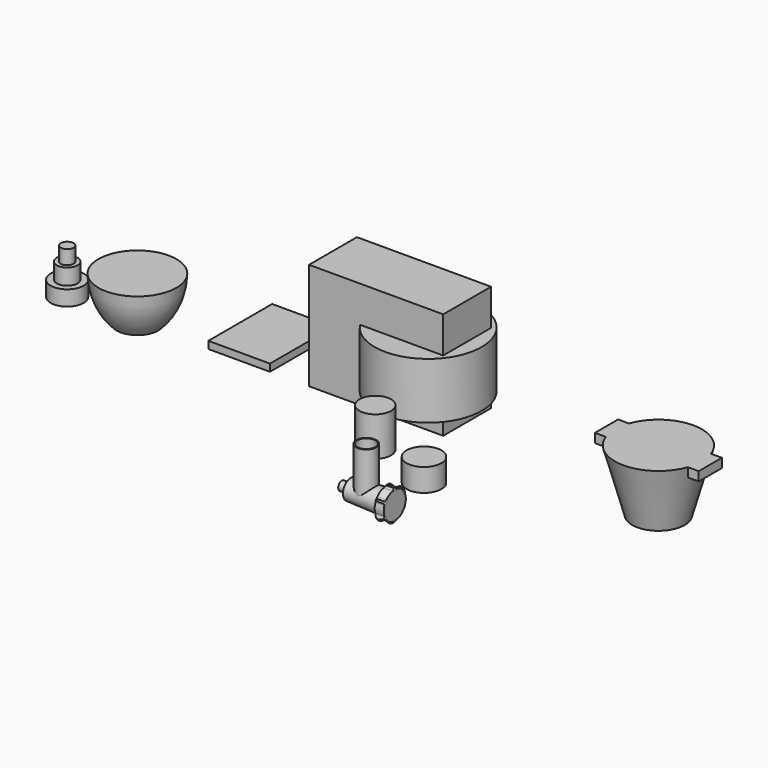
from build123d import *

# Parameters (mm, degrees)
F0_W          = 170
F0_H          = 220
F1_DEPTH      = 20
F2_W          = 370
F2_H          = 165
F3_DEPTH      = 40
F5_DEPTH      = 155
F6_W          = 370
F6_H          = 165
F7_DEPTH      = 100
F10_W         = 30
F10_H         = 80
F11_DEPTH     = 25
F12_R         = 43.5
F13_DEPTH     = 108
F14_R         = 48
F15_DEPTH     = 63
F16_R         = 27.5
F19_R         = 31
F22_DEPTH     = 25
F23_R         = 12.49999
F24_T4_DEPTH  = 46.1160280669
F24_S5_R      = 12.49999
F24_T6_DEPTH  = 25
F24_T10_DEPTH = 46.1160280669
F24_S11_R     = 12.49999
F24_T12_DEPTH = 25
F24_T16_DEPTH = 46.1160280669
F24_S17_R     = 12.49999
F24_T18_DEPTH = 25
F24_T22_DEPTH = 46.1160280669
F24_S23_R     = 12.49999
F24_T24_DEPTH = 25
F24_T28_DEPTH = 46.1160280669
F24_S29_R     = 12.49999
F24_T30_DEPTH = 25
F24_T34_DEPTH = 46.1160280669
F24_S35_R     = 12.49999
F24_T36_DEPTH = 25
F24_T40_DEPTH = 46.1160280669
F24_S41_R     = 12.49999
F24_T42_DEPTH = 25
F24_T46_DEPTH = 46.1160280669
F24_S47_R     = 12.49999
F24_T48_DEPTH = 25
F24_T52_DEPTH = 46.1160280669
F24_S53_R     = 12.49999
F24_T54_DEPTH = 25
F24_T58_DEPTH = 46.1160280669
F24_S59_R     = 12.49999
F24_T60_DEPTH = 25
F24_T64_DEPTH = 46.1160280669
F24_S65_R     = 12.49999
F24_T66_DEPTH = 25
F24_T70_DEPTH = 46.1160280669
F24_S71_R     = 12.49999
F24_T72_DEPTH = 25
F25_R         = 12.5
F26_DEPTH     = 25
F27_R         = 27.5
F27_R_2       = 25
F28_DEPTH     = 124


# Not quite as in the source:
# - a fillet or chamfer that OpenCascade refuses, or shapes differently, is made with other operations: its cross-section is extruded or revolved along the edge and cut away or added
# - a fillet or chamfer is up to 0.001 mm smaller than in the source, because OpenCascade refuses the exact size


with BuildPart() as f1:
    # F0 (on Top) → F1 (new body)
    with BuildSketch(Plane.XY):
        with Locations((-562.7675076718, 110)):
            Rectangle(F0_W, F0_H)
    extrude(amount=F1_DEPTH)


with BuildPart() as f3:
    # F2 (on Top) → F3 (new body)
    with BuildSketch(Plane.XY):
        with Locations((-185, 82.5)):
            Rectangle(F2_W, F2_H)
    extrude(amount=F3_DEPTH)

    # F4 (on face) → F5 (join)
    with BuildSketch(Plane.XY.offset(40)):
        with BuildLine():
            Line((-370, 0), (-229.7701926064, 0))
            ThreePointArc((-229.7701926064, 0), (40, 82.5), (-229.7701926064, 165))
            Line((-229.7701926064, 165), (-370, 165))
            Line((-370, 165), (-370, 0))
        make_face()
    extrude(amount=F5_DEPTH)

    # F6 (on face) → F7 (join)
    with BuildSketch(Plane.XY.offset(195)):
        with Locations((-185, 82.5)):
            Rectangle(F6_W, F6_H)
    extrude(amount=F7_DEPTH)


with BuildPart() as f9:
    # F8 (on Front) → F9 (revolve)
    with BuildSketch(Plane.XZ):
        Polygon((593.6409032087, 170), (593.6409032087, 0), (666.1409032087, 0), (713.6409032087, 170), align=None)
    revolve(axis=Axis((593.6409032087, 0, 85), (0, 0, 1)))

    # F10 (on face) → F11 (join)
    with BuildSketch(Plane.XY.offset(170)):
        with Locations((465.5038182188, 0)):
            Rectangle(F10_W, F10_H)
        with Locations((721.7779881985, 0)):
            Rectangle(F10_W, F10_H)
    extrude(amount=-F11_DEPTH)


with BuildPart() as f13:
    # F12 (on Top) → F13 (new body)
    with BuildSketch(Plane.XY):
        with Locations((-74.1944685578, -141.4187550545)):
            Circle(F12_R)
    extrude(amount=F13_DEPTH)


with BuildPart() as f15:
    # F14 (on Top) → F15 (new body)
    with BuildSketch(Plane.XY):
        with Locations((104.2551547289, -196.5236961842)):
            Circle(F14_R)
    extrude(amount=F15_DEPTH)


with BuildPart() as f20:
    # F16 (on Right) → F20 section 0
    with BuildSketch(Plane.YZ):
        with Locations((-318.2184583697, 0)):
            Circle(F16_R)
    # F19 (on offset) → F20 section 1
    with BuildSketch(Plane.YZ.offset(96)):
        with Locations((-318.2184583697, 0)):
            Circle(F19_R)
    loft()

    # F21 (on face) → F22 (join)
    with BuildSketch(Plane.YZ.offset(96)):
        with BuildLine():
            Line((-320.7184583697, 46.9176739793), (-320.7184583697, 37.9176739793))
            ThreePointArc((-320.7184583697, 37.9176739793), (-337.2184583697, 32.9089653438), (-349.8061272882, 21.1239004991))
            Line((-349.8061272882, 21.1239004991), (-357.6003559222, 25.6239004991))
            Line((-357.6003559222, 25.6239004991), (-360.1003559222, 21.2937734802))
            Line((-360.1003559222, 21.2937734802), (-352.3061272882, 16.7937734802))
            ThreePointArc((-352.3061272882, 16.7937734802), (-356.2184583697, 0), (-352.3061272882, -16.7937734802))
            Line((-352.3061272882, -16.7937734802), (-360.1003559222, -21.2937734802))
            Line((-360.1003559222, -21.2937734802), (-357.6003559222, -25.6239004991))
            Line((-357.6003559222, -25.6239004991), (-349.8061272882, -21.1239004991))
            ThreePointArc((-349.8061272882, -21.1239004991), (-337.2184583697, -32.9089653438), (-320.7184583697, -37.9176739793))
            Line((-320.7184583697, -37.9176739793), (-320.7184583697, -46.9176739793))
            Line((-320.7184583697, -46.9176739793), (-315.7184583697, -46.9176739793))
            Line((-315.7184583697, -46.9176739793), (-315.7184583697, -37.9176739793))
            ThreePointArc((-315.7184583697, -37.9176739793), (-299.2184583697, -32.9089653438), (-286.6307894512, -21.1239004991))
            Line((-286.6307894512, -21.1239004991), (-278.8365608172, -25.6239004991))
            Line((-278.8365608172, -25.6239004991), (-276.3365608172, -21.2937734802))
            Line((-276.3365608172, -21.2937734802), (-284.1307894512, -16.7937734802))
            ThreePointArc((-284.1307894512, -16.7937734802), (-280.2184583697, 0), (-284.1307894512, 16.7937734802))
            Line((-284.1307894512, 16.7937734802), (-276.3365608172, 21.2937734802))
            Line((-276.3365608172, 21.2937734802), (-278.8365608172, 25.6239004991))
            Line((-278.8365608172, 25.6239004991), (-286.6307894512, 21.1239004991))
            ThreePointArc((-286.6307894512, 21.1239004991), (-299.2184583697, 32.9089653438), (-315.7184583697, 37.9176739793))
            Line((-315.7184583697, 37.9176739793), (-315.7184583697, 46.9176739793))
            Line((-315.7184583697, 46.9176739793), (-320.7184583697, 46.9176739793))
        make_face()
    extrude(amount=F22_DEPTH)

    # F23 (radius 12.5 in the source; OpenCascade refuses exactly that, so slightly less here)
    f23_edges = [f20.edges().sort_by_distance(p)[0] for p in [
        (96, -358.850356, 23.458837),
        (121, -358.850356, 23.458837),
        (96, -358.850356, -23.458837),
        (121, -358.850356, -23.458837),
        (121, -318.218458, -46.917674),
        (96, -318.218458, -46.917674),
        (96, -277.586561, -23.458837),
        (121, -277.586561, -23.458837),
        (96, -277.586561, 23.458837),
        (121, -277.586561, 23.458837),
        (96, -318.218458, 46.917674),
        (121, -318.218458, 46.917674),
    ]]
    fillet(f23_edges, radius=F23_R)

    # F24: fillet of radius 5 on 12 edges, made by hand


with BuildPart() as f24_tool2:
    # F24_s3 → F24_t4 (new body)
    with BuildSketch(Plane.YZ.offset(85.4419859665)):
        with BuildLine():
            ThreePointArc((-353.9369352588, -12.9688244926), (-353.9389410675, -16.3871873128), (-356.1367348495, -19.0053757869))
            Line((-356.1367348495, -19.0053757869), (-352.3061272882, -16.7937734802))
            ThreePointArc((-352.3061272882, -16.7937734802), (-353.1738879454, -14.9036218142), (-353.9369352588, -12.9688244926))
        make_face()
    extrude(amount=F24_T4_DEPTH)

    # F24_s5 → F24_t6 (intersect, symmetric)
    with BuildSketch(Plane(origin=(0, -81.65, 141.421948438), x_dir=(1, 0, 0), z_dir=(0, 0.5, -0.8660254038))):
        with Locations((108.50001, 310.0029528806)):
            Circle(F24_S5_R)
    extrude(amount=F24_T6_DEPTH, both=True, mode=Mode.INTERSECT)


with BuildPart() as f20_1:
    add(f20.part)

    # F24_t1: union F24_tool2
    add(f24_tool2.part)


with BuildPart() as f24_tool8:
    # F24_s9 → F24_t10 (new body)
    with BuildSketch(Plane.YZ.offset(85.4419859665)):
        with BuildLine():
            ThreePointArc((-353.9369352588, 12.9688244926), (-353.9389410675, 16.3871873128), (-356.1367348495, 19.0053757869))
            Line((-356.1367348495, 19.0053757869), (-352.3061272882, 16.7937734802))
            ThreePointArc((-352.3061272882, 16.7937734802), (-353.1738879454, 14.9036218142), (-353.9369352588, 12.9688244926))
        make_face()
    extrude(amount=F24_T10_DEPTH)

    # F24_s11 → F24_t12 (intersect, symmetric)
    with BuildSketch(Plane(origin=(0, -81.65, -141.421948438), x_dir=(1, 0, 0), z_dir=(0, -0.5, -0.8660254038))):
        with Locations((108.50001, 310.0029528806)):
            Circle(F24_S11_R)
    extrude(amount=F24_T12_DEPTH, both=True, mode=Mode.INTERSECT)


with BuildPart() as f20_2:
    add(f20_1.part)

    # F24_t7: union F24_tool8
    add(f24_tool8.part)


with BuildPart() as f24_tool14:
    # F24_s15 → F24_t16 (new body)
    with BuildSketch(Plane.YZ.offset(85.4419859665)):
        with BuildLine():
            ThreePointArc((-347.3090282821, 24.4486961242), (-350.2704202281, 22.7412517953), (-353.6367348495, 23.3355028058))
            Line((-353.6367348495, 23.3355028058), (-349.8061272882, 21.1239004991))
            ThreePointArc((-349.8061272882, 21.1239004991), (-348.6030882571, 22.8204791056), (-347.3090282821, 24.4486961242))
        make_face()
    extrude(amount=F24_T16_DEPTH)

    # F24_s17 → F24_t18 (intersect, symmetric)
    with BuildSketch(Plane(origin=(0, -77.75, -134.6669502885), x_dir=(1, 0, 0), z_dir=(0, -0.5, -0.8660254038))):
        with Locations((108.50001, 310.0029528806)):
            Circle(F24_S17_R)
    extrude(amount=F24_T18_DEPTH, both=True, mode=Mode.INTERSECT)


with BuildPart() as f20_3:
    add(f20_2.part)

    # F24_t13: union F24_tool14
    add(f24_tool14.part)


with BuildPart() as f24_tool20:
    # F24_s21 → F24_t22 (new body)
    with BuildSketch(Plane.YZ.offset(85.4419859665)):
        with BuildLine():
            ThreePointArc((-320.7184583697, 42.3408785927), (-321.8869792091, 39.1284391081), (-324.8463653464, 37.4175206168))
            ThreePointArc((-324.8463653464, 37.4175206168), (-322.789258058, 37.7241009198), (-320.7184583697, 37.9176739793))
            Line((-320.7184583697, 37.9176739793), (-320.7184583697, 42.3408785927))
        make_face()
    extrude(amount=F24_T22_DEPTH)

    # F24_s23 → F24_t24 (intersect, symmetric)
    with BuildSketch(Plane.XZ.offset(322.8)):
        with Locations((108.50001, 34.4176839793)):
            Circle(F24_S23_R)
    extrude(amount=F24_T24_DEPTH, both=True, mode=Mode.INTERSECT)


with BuildPart() as f20_4:
    add(f20_3.part)

    # F24_t19: union F24_tool20
    add(f24_tool20.part)


with BuildPart() as f24_tool26:
    # F24_s27 → F24_t28 (new body)
    with BuildSketch(Plane.YZ.offset(85.4419859665)):
        with BuildLine():
            ThreePointArc((-315.7184583697, 42.3408785927), (-314.5499375303, 39.1284391081), (-311.590551393, 37.4175206168))
            ThreePointArc((-311.590551393, 37.4175206168), (-313.6476586814, 37.7241009198), (-315.7184583697, 37.9176739793))
            Line((-315.7184583697, 37.9176739793), (-315.7184583697, 42.3408785927))
        make_face()
    extrude(amount=F24_T28_DEPTH)

    # F24_s29 → F24_t30 (intersect, symmetric)
    with BuildSketch(Plane.XZ.offset(313.7)):
        with Locations((108.50001, 34.4176839793)):
            Circle(F24_S29_R)
    extrude(amount=F24_T30_DEPTH, both=True, mode=Mode.INTERSECT)


with BuildPart() as f20_5:
    add(f20_4.part)

    # F24_t25: union F24_tool26
    add(f24_tool26.part)


with BuildPart() as f24_tool32:
    # F24_s33 → F24_t34 (new body)
    with BuildSketch(Plane.YZ.offset(85.4419859665)):
        with BuildLine():
            ThreePointArc((-289.1278884573, 24.4486961242), (-286.1664965113, 22.7412517953), (-282.8001818899, 23.3355028058))
            Line((-282.8001818899, 23.3355028058), (-286.6307894512, 21.1239004991))
            ThreePointArc((-286.6307894512, 21.1239004991), (-287.8338284824, 22.8204791056), (-289.1278884573, 24.4486961242))
        make_face()
    extrude(amount=F24_T34_DEPTH)

    # F24_s35 → F24_t36 (intersect, symmetric)
    with BuildSketch(Plane(origin=(0, -81.35, 140.9023331957), x_dir=(1, 0, 0), z_dir=(0, -0.5, 0.8660254038))):
        with Locations((108.50001, -241.167584922)):
            Circle(F24_S35_R)
    extrude(amount=F24_T36_DEPTH, both=True, mode=Mode.INTERSECT)


with BuildPart() as f20_6:
    add(f20_5.part)

    # F24_t31: union F24_tool32
    add(f24_tool32.part)


with BuildPart() as f24_tool38:
    # F24_s39 → F24_t40 (new body)
    with BuildSketch(Plane.YZ.offset(85.4419859665)):
        with BuildLine():
            ThreePointArc((-282.4999814806, 12.9688244926), (-282.4979756719, 16.3871873128), (-280.3001818899, 19.0053757869))
            Line((-280.3001818899, 19.0053757869), (-284.1307894512, 16.7937734802))
            ThreePointArc((-284.1307894512, 16.7937734802), (-283.2630287941, 14.9036218142), (-282.4999814806, 12.9688244926))
        make_face()
    extrude(amount=F24_T40_DEPTH)

    # F24_s41 → F24_t42 (intersect, symmetric)
    with BuildSketch(Plane(origin=(0, -77.5, 134.2339375866), x_dir=(1, 0, 0), z_dir=(0, -0.5, 0.8660254038))):
        with Locations((108.50001, -241.167584922)):
            Circle(F24_S41_R)
    extrude(amount=F24_T42_DEPTH, both=True, mode=Mode.INTERSECT)


with BuildPart() as f20_7:
    add(f20_6.part)

    # F24_t37: union F24_tool38
    add(f24_tool38.part)


with BuildPart() as f24_tool44:
    # F24_s45 → F24_t46 (new body)
    with BuildSketch(Plane.YZ.offset(85.4419859665)):
        with BuildLine():
            ThreePointArc((-282.4999814806, -12.9688244926), (-282.4979756719, -16.3871873128), (-280.3001818899, -19.0053757869))
            Line((-280.3001818899, -19.0053757869), (-284.1307894512, -16.7937734802))
            ThreePointArc((-284.1307894512, -16.7937734802), (-283.2630287941, -14.9036218142), (-282.4999814806, -12.9688244926))
        make_face()
    extrude(amount=F24_T46_DEPTH)

    # F24_s47 → F24_t48 (intersect, symmetric)
    with BuildSketch(Plane(origin=(0, -77.5, -134.2339375866), x_dir=(1, 0, 0), z_dir=(0, 0.5, 0.8660254038))):
        with Locations((108.50001, -241.167584922)):
            Circle(F24_S47_R)
    extrude(amount=F24_T48_DEPTH, both=True, mode=Mode.INTERSECT)


with BuildPart() as f20_8:
    add(f20_7.part)

    # F24_t43: union F24_tool44
    add(f24_tool44.part)


with BuildPart() as f24_tool50:
    # F24_s51 → F24_t52 (new body)
    with BuildSketch(Plane.YZ.offset(85.4419859665)):
        with BuildLine():
            ThreePointArc((-289.1278884573, -24.4486961242), (-286.1664965113, -22.7412517953), (-282.8001818899, -23.3355028058))
            Line((-282.8001818899, -23.3355028058), (-286.6307894512, -21.1239004991))
            ThreePointArc((-286.6307894512, -21.1239004991), (-287.8338284824, -22.8204791056), (-289.1278884573, -24.4486961242))
        make_face()
    extrude(amount=F24_T52_DEPTH)

    # F24_s53 → F24_t54 (intersect, symmetric)
    with BuildSketch(Plane(origin=(0, -81.35, -140.9023331957), x_dir=(1, 0, 0), z_dir=(0, 0.5, 0.8660254038))):
        with Locations((108.50001, -241.167584922)):
            Circle(F24_S53_R)
    extrude(amount=F24_T54_DEPTH, both=True, mode=Mode.INTERSECT)


with BuildPart() as f20_9:
    add(f20_8.part)

    # F24_t49: union F24_tool50
    add(f24_tool50.part)


with BuildPart() as f24_tool56:
    # F24_s57 → F24_t58 (new body)
    with BuildSketch(Plane.YZ.offset(85.4419859665)):
        with BuildLine():
            ThreePointArc((-311.590551393, -37.4175206168), (-314.5499375303, -39.1284391081), (-315.7184583697, -42.3408785927))
            Line((-315.7184583697, -42.3408785927), (-315.7184583697, -37.9176739793))
            ThreePointArc((-315.7184583697, -37.9176739793), (-313.6476586814, -37.7241009198), (-311.590551393, -37.4175206168))
        make_face()
    extrude(amount=F24_T58_DEPTH)

    # F24_s59 → F24_t60 (intersect, symmetric)
    with BuildSketch(Plane.XZ.offset(313.7)):
        with Locations((108.50001, -34.4176839793)):
            Circle(F24_S59_R)
    extrude(amount=F24_T60_DEPTH, both=True, mode=Mode.INTERSECT)


with BuildPart() as f20_10:
    add(f20_9.part)

    # F24_t55: union F24_tool56
    add(f24_tool56.part)


with BuildPart() as f24_tool62:
    # F24_s63 → F24_t64 (new body)
    with BuildSketch(Plane.YZ.offset(85.4419859665)):
        with BuildLine():
            ThreePointArc((-324.8463653464, -37.4175206168), (-321.8869792091, -39.1284391081), (-320.7184583697, -42.3408785927))
            Line((-320.7184583697, -42.3408785927), (-320.7184583697, -37.9176739793))
            ThreePointArc((-320.7184583697, -37.9176739793), (-322.789258058, -37.7241009198), (-324.8463653464, -37.4175206168))
        make_face()
    extrude(amount=F24_T64_DEPTH)

    # F24_s65 → F24_t66 (intersect, symmetric)
    with BuildSketch(Plane.XZ.offset(322.8)):
        with Locations((108.50001, -34.4176839793)):
            Circle(F24_S65_R)
    extrude(amount=F24_T66_DEPTH, both=True, mode=Mode.INTERSECT)


with BuildPart() as f20_11:
    add(f20_10.part)

    # F24_t61: union F24_tool62
    add(f24_tool62.part)


with BuildPart() as f24_tool68:
    # F24_s69 → F24_t70 (new body)
    with BuildSketch(Plane.YZ.offset(85.4419859665)):
        with BuildLine():
            ThreePointArc((-347.3090282821, -24.4486961242), (-350.2704202281, -22.7412517953), (-353.6367348495, -23.3355028058))
            Line((-353.6367348495, -23.3355028058), (-349.8061272882, -21.1239004991))
            ThreePointArc((-349.8061272882, -21.1239004991), (-348.6030882571, -22.8204791056), (-347.3090282821, -24.4486961242))
        make_face()
    extrude(amount=F24_T70_DEPTH)

    # F24_s71 → F24_t72 (intersect, symmetric)
    with BuildSketch(Plane(origin=(0, -77.75, 134.6669502885), x_dir=(1, 0, 0), z_dir=(0, 0.5, -0.8660254038))):
        with Locations((108.50001, 310.0029528806)):
            Circle(F24_S71_R)
    extrude(amount=F24_T72_DEPTH, both=True, mode=Mode.INTERSECT)


with BuildPart() as f20_12:
    add(f20_11.part)

    # F24_t67: union F24_tool68
    add(f24_tool68.part)

    # F25 (on face) → F26 (join)
    with BuildSketch(Plane(origin=(0, 0, 0), x_dir=(0, -1, 0), z_dir=(-1, 0, 0))):
        with Locations((318.2184583697, 0)):
            Circle(F25_R)
    extrude(amount=F26_DEPTH)

    # F27 (on Top) → F28 (join)
    with BuildSketch(Plane.XY):
        with Locations((42.5, -318.2184583697)):
            Circle(F27_R)
        with Locations((42.5, -318.2184583697)):
            Circle(F27_R_2, mode=Mode.SUBTRACT)
    extrude(amount=F28_DEPTH)


with BuildPart() as f30:
    # F29 (on Front) → F30 (revolve)
    with BuildSketch(Plane.XZ):
        with BuildLine():
            Line((-900.9126839638, 0), (-843.4126839638, 0))
            Line((-843.4126839638, 0), (-843.4126839638, 120))
            Line((-843.4126839638, 120), (-950.9126839638, 120))
            ThreePointArc((-950.9126839638, 120), (-937.730736053, 55.0758116295), (-900.9126839638, 0))
        make_face()
    revolve(axis=Axis((-843.4126839638, 0, 60), (0, 0, -1)))


with BuildPart() as f32:
    # F31 (on Front) → F32 (revolve)
    with BuildSketch(Plane.XZ):
        Polygon((-1082.6759468684, 42), (-1082.6759468684, 0), (-1037.1759468684, 0), (-1037.1759468684, 125), (-1054.6759468684, 125), (-1054.6759468684, 86), (-1065.6759468684, 86), (-1065.6759468684, 42), align=None)
    revolve(axis=Axis((-1037.1759468684, 0, 62.5), (0, 0, -1)))


solid = Compound([f1.part, f3.part, f9.part, f13.part, f15.part, f20_12.part, f30.part, f32.part])
